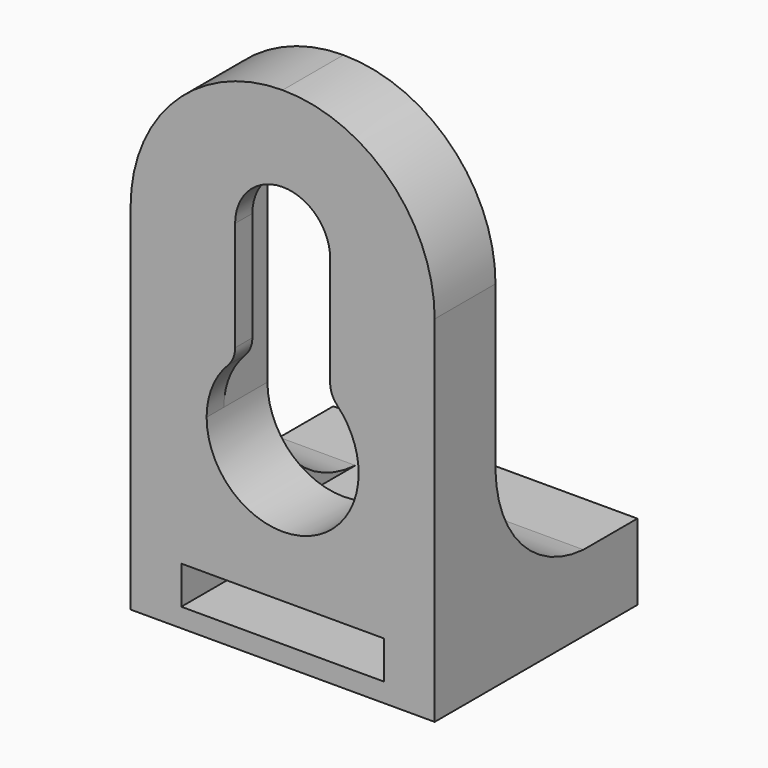
from build123d import *

# Parameters (mm, degrees)
F0_W      = 30.48
F0_H      = 50.8
F2_DEPTH  = 7.62
F3_DEPTH  = 7.62
F4_DEPTH  = 5.461
F5_W      = 30.48
F5_H      = 7.62
F6_DEPTH  = 17.78
F8_DEPTH  = 7.62
F10_DEPTH = 7.62
F11_W     = 20.32
F11_H     = 3.81
F12_DEPTH = 6.35
F13_R     = 15.23999
F14_R     = 2.54


# Not quite as in the source:
# - a fillet or chamfer is up to 0.001 mm smaller than in the source, because OpenCascade refuses the exact size


with BuildPart() as f2:
    # F0 (on Front) → F2 (new body)
    with BuildSketch(Plane.XZ):
        Rectangle(F0_W, F0_H)
    extrude(amount=F2_DEPTH)

    # F1 (on face) → F3 (cut)
    with BuildSketch(Plane.XZ):
        with BuildLine():
            Line((4.7625, 0), (4.7625, 12.0856394065))
            ThreePointArc((4.7625, 12.0856394065), (0, 16.8481394065), (-4.7625, 12.0856394065))
            Line((-4.7625, 12.0856394065), (-4.7625, 0))
            ThreePointArc((-4.7625, 0), (-6.8685751798, -2.6488038051), (-7.62, -5.9483605935))
            ThreePointArc((-7.62, -5.9483605935), (0, -13.5683605935), (7.62, -5.9483605935))
            ThreePointArc((7.62, -5.9483605935), (6.8685751798, -2.6488038051), (4.7625, 0))
        make_face()
    extrude(amount=F3_DEPTH, mode=Mode.SUBTRACT)

    # F1 (on face) → F4 (cut)
    with BuildSketch(Plane.XZ):
        with BuildLine():
            Line((4.7625, 0), (4.7625, 12.0856394065))
            ThreePointArc((4.7625, 12.0856394065), (0, 16.8481394065), (-4.7625, 12.0856394065))
            Line((-4.7625, 12.0856394065), (-4.7625, 0))
            ThreePointArc((-4.7625, 0), (-6.8685751798, -2.6488038051), (-7.62, -5.9483605935))
            ThreePointArc((-7.62, -5.9483605935), (0, -13.5683605935), (7.62, -5.9483605935))
            ThreePointArc((7.62, -5.9483605935), (6.8685751798, -2.6488038051), (4.7625, 0))
        make_face()
        with BuildLine():
            ThreePointArc((-4.7625, 12.0856394065), (0, 16.8481394065), (4.7625, 12.0856394065))
            Line((4.7625, 12.0856394065), (4.7625, 0))
            ThreePointArc((4.7625, 0), (6.8685751798, -2.6488038051), (7.62, -5.9483605935))
            Line((7.62, -5.9483605935), (7.62, 12.0856394065))
            ThreePointArc((7.62, 12.0856394065), (0, 19.7056394065), (-7.62, 12.0856394065))
            Line((-7.62, 12.0856394065), (-7.62, -5.9483605935))
            ThreePointArc((-7.62, -5.9483605935), (-6.8685751798, -2.6488038051), (-4.7625, 0))
            Line((-4.7625, 0), (-4.7625, 12.0856394065))
        make_face()
    extrude(amount=F4_DEPTH, mode=Mode.SUBTRACT)

    # F5 (on face) → F6 (join)
    with BuildSketch(Plane(origin=(0, 0, 0), x_dir=(-1, 0, 0), z_dir=(0, 1, 0))):
        with Locations((0, -21.59)):
            Rectangle(F5_W, F5_H)
    extrude(amount=F6_DEPTH)

    # F7 (on face) → F8 (join)
    with BuildSketch(Plane.YZ.offset(15.24)):
        with BuildLine():
            ThreePointArc((11.0238203779, -17.78), (3.2923822905, -14.1798622678), (0, -6.3124392182))
            Line((0, -6.3124392182), (0, -17.78))
            Line((0, -17.78), (11.0238203779, -17.78))
        make_face()
    extrude(amount=-F8_DEPTH)

    # F9 (on face) → F10 (join)
    with BuildSketch(Plane(origin=(-15.24, 0, 0), x_dir=(0, -1, 0), z_dir=(-1, 0, 0))):
        with BuildLine():
            Line((-11.0238286, -17.78), (0, -17.78))
            Line((0, -17.78), (0, -5.9952606229))
            ThreePointArc((0, -5.9952606229), (-3.1855434206, -14.0637933146), (-11.0238286, -17.78))
        make_face()
    extrude(amount=-F10_DEPTH)

    # F11 (on face) → F12 (cut)
    with BuildSketch(Plane.XZ.offset(7.62)):
        with Locations((0, -21.59)):
            Rectangle(F11_W, F11_H)
    extrude(amount=-F12_DEPTH, mode=Mode.SUBTRACT)

    # F13 (radius 15.24 in the source; OpenCascade refuses exactly that, so slightly less here)
    f13_edges = [f2.edges().sort_by_distance(p)[0] for p in [
        (15.24, -3.81, 25.4),
        (-15.24, -3.81, 25.4),
    ]]
    fillet(f13_edges, radius=F13_R)

    # F14
    f14_edges = [f2.edges().sort_by_distance(p)[0] for p in [
        (4.7625, -6.5405, 0),
        (-4.7625, -6.5405, 0),
    ]]
    fillet(f14_edges, radius=F14_R)


solid = f2.part
